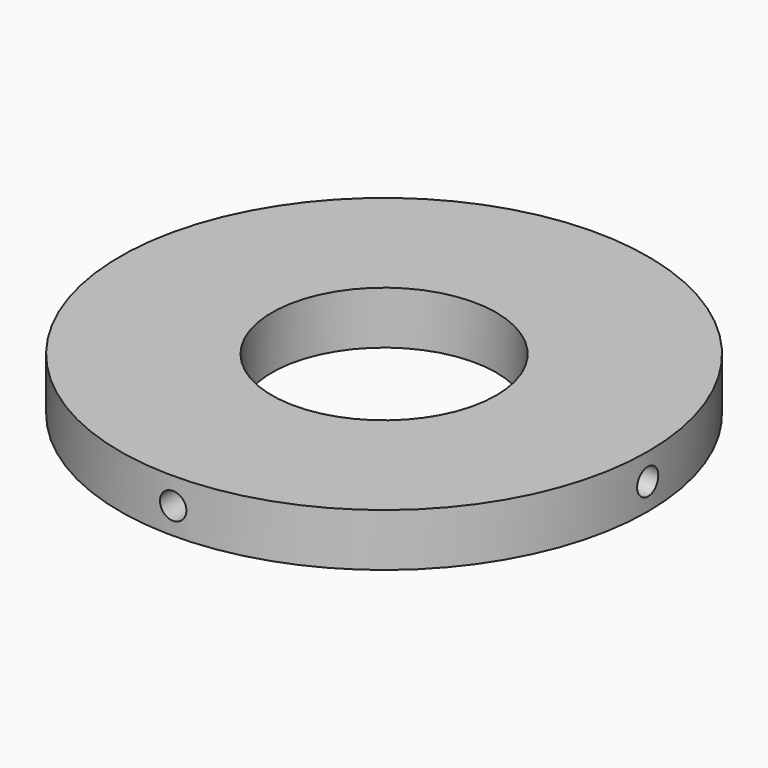
from build123d import *

# Parameters (mm, degrees)
F0_R      = 20
F0_R_2    = 8.5
F1_DEPTH  = 2
F4_D      = 2
F4_DEPTH  = 3
F4_TIP    = 0.600860619
F7_D      = 2
F7_DEPTH  = 3
F7_TIP    = 0.600860619
F10_D     = 2
F10_DEPTH = 3
F10_TIP   = 0.600860619
F13_D     = 2
F13_DEPTH = 3
F13_TIP   = 0.600860619


with BuildPart() as f1:
    # F0 (on Top) → F1 (new body, symmetric)
    with BuildSketch(Plane.XY):
        Circle(F0_R)
        Circle(F0_R_2, mode=Mode.SUBTRACT)
    extrude(amount=F1_DEPTH, both=True)

    # F4 (one way)
    with BuildSketch(Plane.YZ.offset(20)):
        with Locations((0, 0)):
            Circle(F4_D / 2)
    extrude(amount=-F4_DEPTH, mode=Mode.SUBTRACT)
    with Locations(Plane.YZ.offset(20)):
        with Locations((0, 0)):
            with Locations((0, 0, -(F4_DEPTH + F4_TIP / 2))):  # 118° drill point
                Cone(0, F4_D / 2, F4_TIP, mode=Mode.SUBTRACT)

    # F7 (one way)
    with BuildSketch(Plane(origin=(-20, 0, 0), x_dir=(0, 1, 0), z_dir=(-1, 0, 0))):
        with Locations((0, 0)):
            Circle(F7_D / 2)
    extrude(amount=-F7_DEPTH, mode=Mode.SUBTRACT)
    with Locations(Plane(origin=(-20, 0, 0), x_dir=(0, 1, 0), z_dir=(-1, 0, 0))):
        with Locations((0, 0)):
            with Locations((0, 0, -(F7_DEPTH + F7_TIP / 2))):  # 118° drill point
                Cone(0, F7_D / 2, F7_TIP, mode=Mode.SUBTRACT)

    # F10 (one way)
    with BuildSketch(Plane.XZ.offset(20)):
        with Locations((0, 0)):
            Circle(F10_D / 2)
    extrude(amount=-F10_DEPTH, mode=Mode.SUBTRACT)
    with Locations(Plane.XZ.offset(20)):
        with Locations((0, 0)):
            with Locations((0, 0, -(F10_DEPTH + F10_TIP / 2))):  # 118° drill point
                Cone(0, F10_D / 2, F10_TIP, mode=Mode.SUBTRACT)

    # F13 (one way)
    with BuildSketch(Plane(origin=(0, 20, 0), x_dir=(1, 0, 0), z_dir=(0, 1, 0))):
        with Locations((0, 0)):
            Circle(F13_D / 2)
    extrude(amount=-F13_DEPTH, mode=Mode.SUBTRACT)
    with Locations(Plane(origin=(0, 20, 0), x_dir=(1, 0, 0), z_dir=(0, 1, 0))):
        with Locations((0, 0)):
            with Locations((0, 0, -(F13_DEPTH + F13_TIP / 2))):  # 118° drill point
                Cone(0, F13_D / 2, F13_TIP, mode=Mode.SUBTRACT)


solid = f1.part
